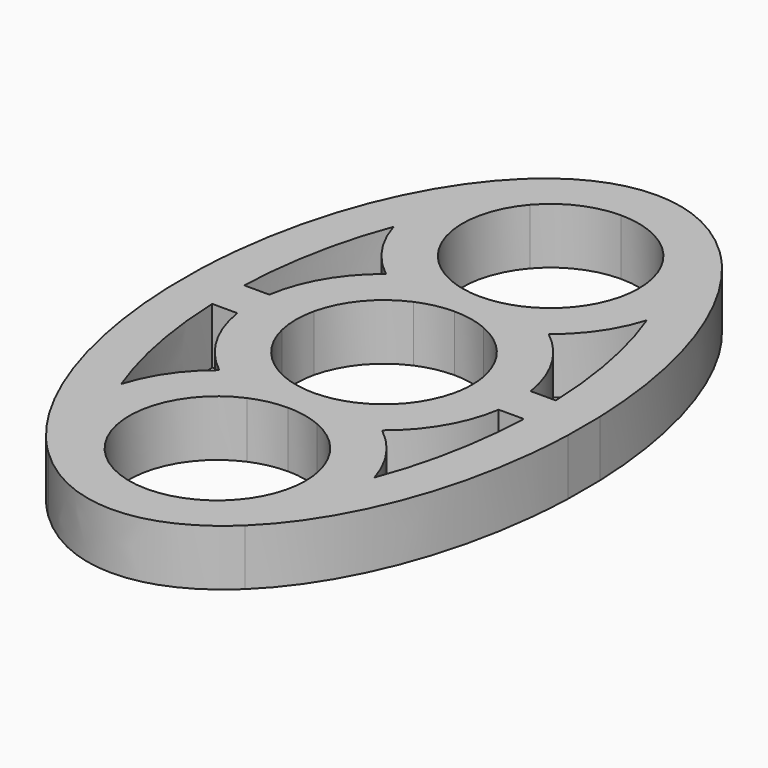
from build123d import *

# Parameters (mm, degrees)
F1_DEPTH = 7


# Not quite as in the source:
# - the dataset's text gives a spline's control points without its knots; the knots are read off the source's solid


with BuildPart() as f1:
    # F0 (on Top) → F1 (new body)
    with BuildSketch(Plane.XY):
        with BuildLine():
            add(Edge.make_bspline(
                [(-12.2865300122, 37.0132275132), (-24.155068252, 25.6273275114), (-24.9567099242, 2.5)],
                knots=[0.5137667663, 0.5137667663, 0.5137667663, 1.5119388208, 1.5119388208, 1.5119388208], degree=2, weights=[1, 0.8780203772, 1]))
            Line((-24.9567099242, 2.5), (-19.453178151, 2.5))
            add(Edge.make_bspline(
                [(-15.8025424867, 21.2534590537), (-16.1608457903, 20.3198762687), (-16.869953541, 18.2823971156), (-17.7856543458, 14.9897380208), (-18.5393237245, 11.414650213), (-19.0884029155, 7.7049435305), (-19.352047015, 4.7083391393), (-19.4358731607, 2.9613993071), (-19.453178151, 2.5)],
                knots=[0.157845185, 0.157845185, 0.157845185, 0.157845185, 0.171875, 0.1875, 0.203125, 0.21875, 0.234375, 0.2399591803, 0.2399591803, 0.2399591803, 0.2399591803], degree=3))
            ThreePointArc((-15.8025424867, 21.2534590537), (-16.1040856287, 29.5928298126), (-12.2865300122, 37.0132275132))
        make_face()
        with BuildLine():
            Line((-19.453178151, 2.5), (-24.9567099242, 2.5))
            Line((-24.9567099242, 2.5), (-24.9567099242, -2.5))
            Line((-24.9567099242, -2.5), (-19.453178151, -2.5))
            add(Edge.make_bspline(
                [(-19.453178151, 2.5), (-19.4600835604, 2.3158825262), (-19.4877799652, 1.485210562), (-19.5095080905, 0), (-19.4877799652, -1.485210562), (-19.4600835604, -2.3158825262), (-19.453178151, -2.5)],
                knots=[0.2399591803, 0.2399591803, 0.2399591803, 0.2399591803, 0.2421875, 0.25, 0.2578125, 0.2600408197, 0.2600408197, 0.2600408197, 0.2600408197], degree=3))
        make_face()
        with BuildLine():
            Line((-19.453178151, -2.5), (-24.9567099242, -2.5))
            add(Edge.make_bspline(
                [(-24.9567099242, -2.5), (-24.155068252, -25.6273275114), (-12.2865300122, -37.0132275132)],
                knots=[1.6296538327, 1.6296538327, 1.6296538327, 2.6278258872, 2.6278258872, 2.6278258872], degree=2, weights=[1, 0.8780203772, 1]))
            ThreePointArc((-12.2865300122, -37.0132275132), (-16.1040856287, -29.5928298126), (-15.8025424867, -21.2534590537))
            add(Edge.make_bspline(
                [(-19.453178151, -2.5), (-19.4358731607, -2.9613993071), (-19.352047015, -4.7083391393), (-19.0884029155, -7.7049435305), (-18.5393237245, -11.414650213), (-17.7856543458, -14.9897380208), (-16.869953541, -18.2823971156), (-16.1608457903, -20.3198762687), (-15.8025424867, -21.2534590537)],
                knots=[0.2600408197, 0.2600408197, 0.2600408197, 0.2600408197, 0.265625, 0.28125, 0.296875, 0.3125, 0.328125, 0.342154815, 0.342154815, 0.342154815, 0.342154815], degree=3))
        make_face()
        with BuildLine():
            add(Edge.make_bspline(
                [(0, 42.5), (-6.5671780891, 42.5), (-12.2865300122, 37.0132275132)],
                knots=[0, 0, 0, 0.5137667663, 0.5137667663, 0.5137667663], degree=2, weights=[1, 0.967186505, 1]))
            ThreePointArc((-12.2865300122, 37.0132275132), (-16.1040856287, 29.5928298126), (-15.8025424867, 21.2534590537))
            add(Edge.make_bspline(
                [(-8.3223566434, 33.1929395869), (-8.7992109435, 32.7452255263), (-9.831903457, 31.6798268662), (-11.1152962392, 30.0683455079), (-12.1705625375, 28.5237462249), (-12.9418479396, 27.2765788333), (-13.6842337818, 25.9505034679), (-14.6253408369, 24.0934250391), (-15.3188374514, 22.5012494774), (-15.7618035271, 21.3596070883), (-15.8025424867, 21.2534590537)],
                knots=[0.0804159275, 0.0804159275, 0.0804159275, 0.0804159275, 0.09375, 0.109375, 0.1171875, 0.125, 0.1328125, 0.140625, 0.15625, 0.157845185, 0.157845185, 0.157845185, 0.157845185], degree=3))
            ThreePointArc((-8.3223566434, 33.1929395869), (-4.5758968817, 36.0030579189), (0, 37))
            ThreePointArc((0, 37), (4.5758968817, 36.0030579189), (8.3223566434, 33.1929395869))
            add(Edge.make_bspline(
                [(15.8025424867, 21.2534590537), (15.7618035271, 21.3596070883), (15.3188374514, 22.5012494774), (14.6253408369, 24.0934250391), (13.6842337818, 25.9505034679), (12.9418479396, 27.2765788333), (12.1705625375, 28.5237462249), (11.1152962392, 30.0683455079), (9.831903457, 31.6798268662), (8.7992109435, 32.7452255263), (8.3223566434, 33.1929395869)],
                knots=[0.842154815, 0.842154815, 0.842154815, 0.842154815, 0.84375, 0.859375, 0.8671875, 0.875, 0.8828125, 0.890625, 0.90625, 0.9195840725, 0.9195840725, 0.9195840725, 0.9195840725], degree=3))
            ThreePointArc((15.8025424867, 21.2534590537), (16.3247044542, 23.6012452221), (16.5, 26))
            ThreePointArc((16.5, 26), (15.4106739827, 31.8958567994), (12.2865300122, 37.0132275132))
            add(Edge.make_bspline(
                [(12.2865300122, 37.0132275132), (6.5671780891, 42.5), (0, 42.5)],
                knots=[5.7694185408, 5.7694185408, 5.7694185408, 6.2831853072, 6.2831853072, 6.2831853072], degree=2, weights=[1, 0.967186505, 1]))
        make_face()
        with BuildLine():
            Line((-16.3095064303, 2.5), (-19.453178151, 2.5))
            add(Edge.make_bspline(
                [(-19.453178151, 2.5), (-19.4600835604, 2.3158825262), (-19.4877799652, 1.485210562), (-19.5095080905, 0), (-19.4877799652, -1.485210562), (-19.4600835604, -2.3158825262), (-19.453178151, -2.5)],
                knots=[0.2399591803, 0.2399591803, 0.2399591803, 0.2399591803, 0.2421875, 0.25, 0.2578125, 0.2600408197, 0.2600408197, 0.2600408197, 0.2600408197], degree=3))
            Line((-19.453178151, -2.5), (-16.3095064303, -2.5))
            ThreePointArc((-16.3095064303, -2.5), (-16.5, 0), (-16.3095064303, 2.5))
        make_face()
        with BuildLine():
            ThreePointArc((-15.8025424867, -21.2534590537), (-16.1040856287, -29.5928298126), (-12.2865300122, -37.0132275132))
            add(Edge.make_bspline(
                [(-12.2865300122, -37.0132275132), (-6.5671782692, -42.4999998273), (-3.868e-07, -42.5)],
                knots=[2.6278258872, 2.6278258872, 2.6278258872, 3.1415926381, 3.1415926381, 3.1415926381], degree=2, weights=[1, 0.967186507, 1]))
            add(Edge.make_bspline(
                [(-3.868e-07, -42.5), (6.5671779091, -42.5000001727), (12.2865300122, -37.0132275132)],
                knots=[3.1415926381, 3.1415926381, 3.1415926381, 3.6553594199, 3.6553594199, 3.6553594199], degree=2, weights=[1, 0.967186503, 1]))
            ThreePointArc((12.2865300122, -37.0132275132), (15.4106739827, -31.8958567994), (16.5, -26))
            ThreePointArc((16.5, -26), (16.3247044542, -23.6012452221), (15.8025424867, -21.2534590537))
            add(Edge.make_bspline(
                [(8.3223566434, -33.1929395869), (8.7992109435, -32.7452255263), (9.831903457, -31.6798268662), (11.1152962392, -30.0683455079), (12.1705625375, -28.5237462249), (12.9418479396, -27.2765788333), (13.6842337818, -25.9505034679), (14.6253408369, -24.0934250391), (15.3188374514, -22.5012494774), (15.7618035271, -21.3596070883), (15.8025424867, -21.2534590537)],
                knots=[0.5804159275, 0.5804159275, 0.5804159275, 0.5804159275, 0.59375, 0.609375, 0.6171875, 0.625, 0.6328125, 0.640625, 0.65625, 0.657845185, 0.657845185, 0.657845185, 0.657845185], degree=3))
            ThreePointArc((8.3223566434, -33.1929395869), (4.5758969132, -36.0030579045), (6.92e-08, -37))
            ThreePointArc((6.92e-08, -37), (-4.5758968503, -36.0030579332), (-8.3223566434, -33.1929395869))
            add(Edge.make_bspline(
                [(-15.8025424867, -21.2534590537), (-15.7618035271, -21.3596070883), (-15.3188374514, -22.5012494774), (-14.6253408369, -24.0934250391), (-13.6842337818, -25.9505034679), (-12.9418479396, -27.2765788333), (-12.1705625375, -28.5237462249), (-11.1152962392, -30.0683455079), (-9.831903457, -31.6798268662), (-8.7992109435, -32.7452255263), (-8.3223566434, -33.1929395869)],
                knots=[0.342154815, 0.342154815, 0.342154815, 0.342154815, 0.34375, 0.359375, 0.3671875, 0.375, 0.3828125, 0.390625, 0.40625, 0.4195840725, 0.4195840725, 0.4195840725, 0.4195840725], degree=3))
        make_face()
        with BuildLine():
            add(Edge.make_bspline(
                [(-8.3223566434, 33.1929395869), (-8.7992109435, 32.7452255263), (-9.831903457, 31.6798268662), (-11.1152962392, 30.0683455079), (-12.1705625375, 28.5237462249), (-12.9418479396, 27.2765788333), (-13.6842337818, 25.9505034679), (-14.6253408369, 24.0934250391), (-15.3188374514, 22.5012494774), (-15.7618035271, 21.3596070883), (-15.8025424867, 21.2534590537)],
                knots=[0.0804159275, 0.0804159275, 0.0804159275, 0.0804159275, 0.09375, 0.109375, 0.1171875, 0.125, 0.1328125, 0.140625, 0.15625, 0.157845185, 0.157845185, 0.157845185, 0.157845185], degree=3))
            ThreePointArc((-15.8025424867, 21.2534590537), (-13.6220001053, 16.6891937443), (-10.1612007165, 13))
            ThreePointArc((-10.1612007165, 13), (-7.4135261595, 14.7407472633), (-4.3777543105, 15.9086538462))
            ThreePointArc((-4.3777543105, 15.9086538462), (-10.7242639818, 23.5525192446), (-8.3223566434, 33.1929395869))
        make_face()
        with BuildLine():
            Line((-10.7121426428, 2.5), (-16.3095064303, 2.5))
            ThreePointArc((-16.3095064303, 2.5), (-16.5, 0), (-16.3095064303, -2.5))
            Line((-16.3095064303, -2.5), (-10.7121426428, -2.5))
            ThreePointArc((-10.7121426428, -2.5), (-11, 0), (-10.7121426428, 2.5))
        make_face()
        with BuildLine():
            ThreePointArc((-10.1612007165, 13), (-14.238577324, 8.3374406018), (-16.3095064303, 2.5))
            Line((-16.3095064303, 2.5), (-10.7121426428, 2.5))
            ThreePointArc((-10.7121426428, 2.5), (-8.4459091649, 7.0474547446), (-4.3777543105, 10.0913461538))
            ThreePointArc((-4.3777543105, 10.0913461538), (-7.4135261595, 11.2592527367), (-10.1612007165, 13))
        make_face()
        with BuildLine():
            ThreePointArc((-10.1612007165, -13), (-13.6220001053, -16.6891937443), (-15.8025424867, -21.2534590537))
            add(Edge.make_bspline(
                [(-15.8025424867, -21.2534590537), (-15.7618035271, -21.3596070883), (-15.3188374514, -22.5012494774), (-14.6253408369, -24.0934250391), (-13.6842337818, -25.9505034679), (-12.9418479396, -27.2765788333), (-12.1705625375, -28.5237462249), (-11.1152962392, -30.0683455079), (-9.831903457, -31.6798268662), (-8.7992109435, -32.7452255263), (-8.3223566434, -33.1929395869)],
                knots=[0.342154815, 0.342154815, 0.342154815, 0.342154815, 0.34375, 0.359375, 0.3671875, 0.375, 0.3828125, 0.390625, 0.40625, 0.4195840725, 0.4195840725, 0.4195840725, 0.4195840725], degree=3))
            ThreePointArc((-8.3223566434, -33.1929395869), (-10.7242639818, -23.5525192446), (-4.3777543105, -15.9086538462))
            ThreePointArc((-4.3777543105, -15.9086538462), (-7.4135261595, -14.7407472633), (-10.1612007165, -13))
        make_face()
        with BuildLine():
            Line((-10.7121426428, -2.5), (-16.3095064303, -2.5))
            ThreePointArc((-16.3095064303, -2.5), (-14.238577324, -8.3374406018), (-10.1612007165, -13))
            ThreePointArc((-10.1612007165, -13), (-7.4135261595, -11.2592527367), (-4.3777543105, -10.0913461538))
            ThreePointArc((-4.3777543105, -10.0913461538), (-8.4459091649, -7.0474547446), (-10.7121426428, -2.5))
        make_face()
        with BuildLine():
            add(Edge.make_bspline(
                [(24.9567099242, 2.5), (24.155068252, 25.6273275114), (12.2865300122, 37.0132275132)],
                knots=[4.7712464863, 4.7712464863, 4.7712464863, 5.7694185408, 5.7694185408, 5.7694185408], degree=2, weights=[1, 0.8780203772, 1]))
            ThreePointArc((12.2865300122, 37.0132275132), (15.4106739827, 31.8958567994), (16.5, 26))
            ThreePointArc((16.5, 26), (16.3247044542, 23.6012452221), (15.8025424867, 21.2534590537))
            add(Edge.make_bspline(
                [(19.453178151, 2.5), (19.4358731607, 2.9613993071), (19.352047015, 4.7083391393), (19.0884029155, 7.7049435305), (18.5393237245, 11.414650213), (17.7856543458, 14.9897380208), (16.869953541, 18.2823971156), (16.1608457903, 20.3198762687), (15.8025424867, 21.2534590537)],
                knots=[0.7600408197, 0.7600408197, 0.7600408197, 0.7600408197, 0.765625, 0.78125, 0.796875, 0.8125, 0.828125, 0.842154815, 0.842154815, 0.842154815, 0.842154815], degree=3))
            Line((19.453178151, 2.5), (24.9567099242, 2.5))
        make_face()
        with BuildLine():
            ThreePointArc((-4.3777543105, 15.9086538462), (-7.4135261595, 14.7407472633), (-10.1612007165, 13))
            ThreePointArc((-10.1612007165, 13), (-7.4135261595, 11.2592527367), (-4.3777543105, 10.0913461538))
            ThreePointArc((-4.3777543105, 10.0913461538), (-2.2355303965, 10.7704412094), (0, 11))
            Line((0, 11), (0, 15))
            ThreePointArc((0, 15), (-2.2355303965, 15.2295587906), (-4.3777543105, 15.9086538462))
        make_face()
        with BuildLine():
            ThreePointArc((16.5, -26), (15.4106739827, -31.8958567994), (12.2865300122, -37.0132275132))
            add(Edge.make_bspline(
                [(12.2865300122, -37.0132275132), (24.155068252, -25.6273275114), (24.9567099242, -2.5)],
                knots=[3.6553594199, 3.6553594199, 3.6553594199, 4.6535314744, 4.6535314744, 4.6535314744], degree=2, weights=[1, 0.8780203772, 1]))
            Line((24.9567099242, -2.5), (19.453178151, -2.5))
            add(Edge.make_bspline(
                [(15.8025424867, -21.2534590537), (16.1608457903, -20.3198762687), (16.869953541, -18.2823971156), (17.7856543458, -14.9897380208), (18.5393237245, -11.414650213), (19.0884029155, -7.7049435305), (19.352047015, -4.7083391393), (19.4358731607, -2.9613993071), (19.453178151, -2.5)],
                knots=[0.657845185, 0.657845185, 0.657845185, 0.657845185, 0.671875, 0.6875, 0.703125, 0.71875, 0.734375, 0.7399591803, 0.7399591803, 0.7399591803, 0.7399591803], degree=3))
            ThreePointArc((15.8025424867, -21.2534590537), (16.3247044542, -23.6012452221), (16.5, -26))
        make_face()
        with BuildLine():
            ThreePointArc((-4.3777543105, -10.0913461538), (-7.4135261595, -11.2592527367), (-10.1612007165, -13))
            ThreePointArc((-10.1612007165, -13), (-7.4135261595, -14.7407472633), (-4.3777543105, -15.9086538462))
            ThreePointArc((-4.3777543105, -15.9086538462), (-2.2355303965, -15.2295587906), (0, -15))
            Line((0, -15), (0, -11))
            ThreePointArc((0, -11), (-2.2355303965, -10.7704412094), (-4.3777543105, -10.0913461538))
        make_face()
        with BuildLine():
            Line((24.9567099242, -2.5), (24.9567099242, 2.5))
            Line((24.9567099242, 2.5), (19.453178151, 2.5))
            add(Edge.make_bspline(
                [(19.453178151, -2.5), (19.4600835604, -2.3158825262), (19.4877799652, -1.485210562), (19.5095080905, 0), (19.4877799652, 1.485210562), (19.4600835604, 2.3158825262), (19.453178151, 2.5)],
                knots=[0.7399591803, 0.7399591803, 0.7399591803, 0.7399591803, 0.7421875, 0.75, 0.7578125, 0.7600408197, 0.7600408197, 0.7600408197, 0.7600408197], degree=3))
            Line((19.453178151, -2.5), (24.9567099242, -2.5))
        make_face()
        with BuildLine():
            add(Edge.make_bspline(
                [(19.453178151, -2.5), (19.4600835604, -2.3158825262), (19.4877799652, -1.485210562), (19.5095080905, 0), (19.4877799652, 1.485210562), (19.4600835604, 2.3158825262), (19.453178151, 2.5)],
                knots=[0.7399591803, 0.7399591803, 0.7399591803, 0.7399591803, 0.7421875, 0.75, 0.7578125, 0.7600408197, 0.7600408197, 0.7600408197, 0.7600408197], degree=3))
            Line((19.453178151, 2.5), (16.3095064303, 2.5))
            ThreePointArc((16.3095064303, 2.5), (16.4523076816, 1.253623528), (16.5, 0))
            ThreePointArc((16.5, 0), (16.4523076816, -1.253623528), (16.3095064303, -2.5))
            Line((16.3095064303, -2.5), (19.453178151, -2.5))
        make_face()
        with BuildLine():
            ThreePointArc((10.1612007165, 13), (13.6220001053, 16.6891937443), (15.8025424867, 21.2534590537))
            add(Edge.make_bspline(
                [(15.8025424867, 21.2534590537), (15.7618035271, 21.3596070883), (15.3188374514, 22.5012494774), (14.6253408369, 24.0934250391), (13.6842337818, 25.9505034679), (12.9418479396, 27.2765788333), (12.1705625375, 28.5237462249), (11.1152962392, 30.0683455079), (9.831903457, 31.6798268662), (8.7992109435, 32.7452255263), (8.3223566434, 33.1929395869)],
                knots=[0.842154815, 0.842154815, 0.842154815, 0.842154815, 0.84375, 0.859375, 0.8671875, 0.875, 0.8828125, 0.890625, 0.90625, 0.9195840725, 0.9195840725, 0.9195840725, 0.9195840725], degree=3))
            ThreePointArc((8.3223566434, 33.1929395869), (10.3088778021, 29.8375823719), (11, 26))
            ThreePointArc((11, 26), (9.1966107185, 19.9649066874), (4.3777543105, 15.9086538462))
            ThreePointArc((4.3777543105, 15.9086538462), (7.4135261595, 14.7407472633), (10.1612007165, 13))
        make_face()
        with BuildLine():
            ThreePointArc((4.3777543105, 15.9086538462), (2.2355303965, 15.2295587906), (0, 15))
            Line((0, 15), (0, 11))
            ThreePointArc((0, 11), (2.2355303965, 10.7704412094), (4.3777543105, 10.0913461538))
            ThreePointArc((4.3777543105, 10.0913461538), (7.4135261595, 11.2592527367), (10.1612007165, 13))
            ThreePointArc((10.1612007165, 13), (7.4135261595, 14.7407472633), (4.3777543105, 15.9086538462))
        make_face()
        with BuildLine():
            Line((16.3095064303, 2.5), (10.7121426428, 2.5))
            ThreePointArc((10.7121426428, 2.5), (10.9277987049, 1.258258902), (11, 0))
            ThreePointArc((11, 0), (10.9277987049, -1.258258902), (10.7121426428, -2.5))
            Line((10.7121426428, -2.5), (16.3095064303, -2.5))
            ThreePointArc((16.3095064303, -2.5), (16.4523076816, -1.253623528), (16.5, 0))
            ThreePointArc((16.5, 0), (16.4523076816, 1.253623528), (16.3095064303, 2.5))
        make_face()
        with BuildLine():
            ThreePointArc((4.3777543105, 10.0913461538), (8.4459091649, 7.0474547446), (10.7121426428, 2.5))
            Line((10.7121426428, 2.5), (16.3095064303, 2.5))
            ThreePointArc((16.3095064303, 2.5), (14.238577324, 8.3374406018), (10.1612007165, 13))
            ThreePointArc((10.1612007165, 13), (7.4135261595, 11.2592527367), (4.3777543105, 10.0913461538))
        make_face()
        with BuildLine():
            add(Edge.make_bspline(
                [(8.3223566434, -33.1929395869), (8.7992109435, -32.7452255263), (9.831903457, -31.6798268662), (11.1152962392, -30.0683455079), (12.1705625375, -28.5237462249), (12.9418479396, -27.2765788333), (13.6842337818, -25.9505034679), (14.6253408369, -24.0934250391), (15.3188374514, -22.5012494774), (15.7618035271, -21.3596070883), (15.8025424867, -21.2534590537)],
                knots=[0.5804159275, 0.5804159275, 0.5804159275, 0.5804159275, 0.59375, 0.609375, 0.6171875, 0.625, 0.6328125, 0.640625, 0.65625, 0.657845185, 0.657845185, 0.657845185, 0.657845185], degree=3))
            ThreePointArc((15.8025424867, -21.2534590537), (13.6220001053, -16.6891937443), (10.1612007165, -13))
            ThreePointArc((10.1612007165, -13), (7.4135261595, -14.7407472633), (4.3777543105, -15.9086538462))
            ThreePointArc((4.3777543105, -15.9086538462), (9.1966107185, -19.9649066874), (11, -26))
            ThreePointArc((11, -26), (10.3088778021, -29.8375823719), (8.3223566434, -33.1929395869))
        make_face()
        with BuildLine():
            Line((0, -11), (0, -15))
            ThreePointArc((0, -15), (2.2355303965, -15.2295587906), (4.3777543105, -15.9086538462))
            ThreePointArc((4.3777543105, -15.9086538462), (7.4135261595, -14.7407472633), (10.1612007165, -13))
            ThreePointArc((10.1612007165, -13), (7.4135261595, -11.2592527367), (4.3777543105, -10.0913461538))
            ThreePointArc((4.3777543105, -10.0913461538), (2.2355303965, -10.7704412094), (0, -11))
        make_face()
        with BuildLine():
            Line((16.3095064303, -2.5), (10.7121426428, -2.5))
            ThreePointArc((10.7121426428, -2.5), (8.4459091649, -7.0474547446), (4.3777543105, -10.0913461538))
            ThreePointArc((4.3777543105, -10.0913461538), (7.4135261595, -11.2592527367), (10.1612007165, -13))
            ThreePointArc((10.1612007165, -13), (14.238577324, -8.3374406018), (16.3095064303, -2.5))
        make_face()
    extrude(amount=F1_DEPTH)


solid = f1.part
